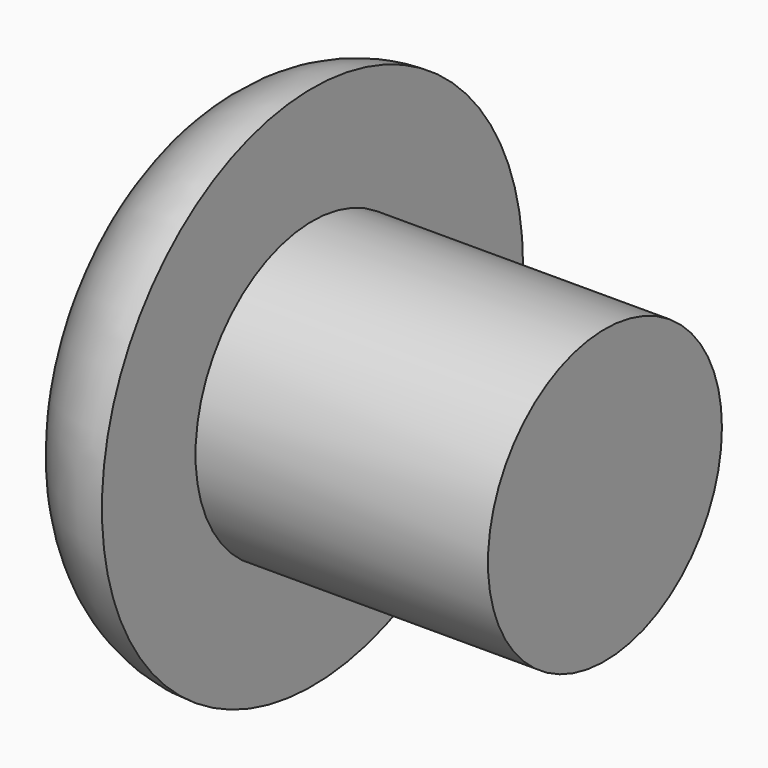
from build123d import *

# Parameters (mm, degrees)
F0_R     = 25
F1_DEPTH = 50
F0_R_2   = 45
F2_DEPTH = 20
F3_R     = 19.99999


# Not quite as in the source:
# - a fillet or chamfer is up to 0.001 mm smaller than in the source, because OpenCascade refuses the exact size


with BuildPart() as f1:
    # F0 (on Right) → F1 (new body)
    with BuildSketch(Plane.YZ):
        Circle(F0_R)
    extrude(amount=F1_DEPTH)


with BuildPart() as f2:
    # F0 (on Right) → F2 (new body)
    with BuildSketch(Plane.YZ):
        Circle(F0_R_2)
        Circle(F0_R, mode=Mode.SUBTRACT)
        Circle(F0_R)
    extrude(amount=-F2_DEPTH)

    # F3 (radius 20 in the source; OpenCascade refuses exactly that, so slightly less here)
    f3_edges = [f2.edges().sort_by_distance(p)[0] for p in [
        (-20, -45, 0),
    ]]
    fillet(f3_edges, radius=F3_R)


solid = Compound([f1.part, f2.part])
